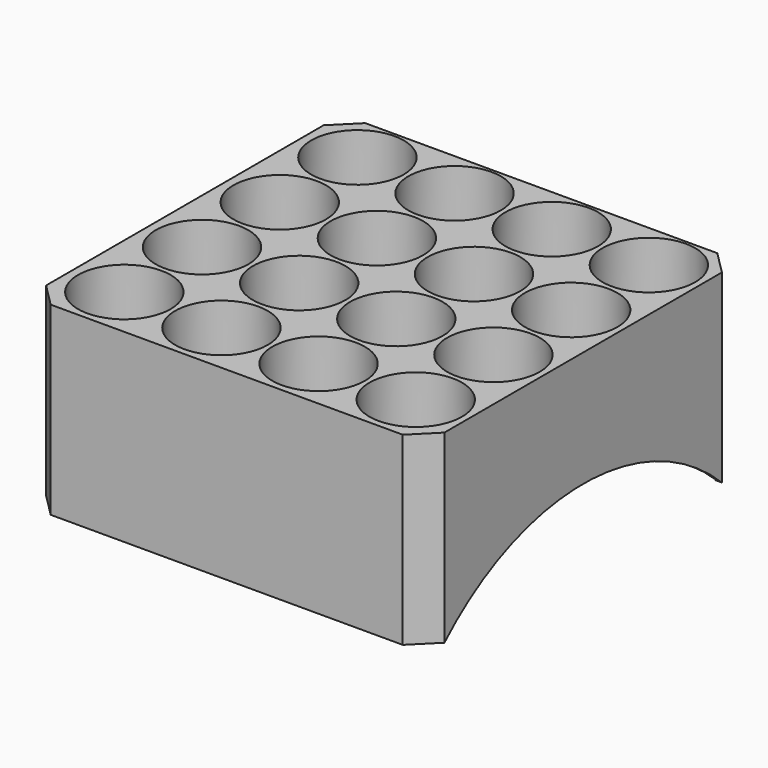
from build123d import *

# Parameters (mm, degrees)
F0_W      = 189
F0_H      = 85
F1_DEPTH  = 40
F2_R      = 10
F3_DEPTH  = 39
F4_W      = 102.8933165297
F4_H      = 85
F5_DEPTH  = 40.001
F6_SIZE   = 5
F8_DEPTH  = 25
F10_DEPTH = 86.1076834703


# Not quite as in the source:
# - a feature names something its author has since deleted; it is built from what else it names


with BuildPart() as f1:
    # F0 (on Top) → F1 (new body)
    with BuildSketch(Plane.XY):
        Rectangle(F0_W, F0_H)
    extrude(amount=F1_DEPTH)

    # F2 (on face) → F3 (cut)
    with BuildSketch(Plane.XY.offset(40)):
        with Locations((-82.6875, 31.875)):
            Circle(F2_R)
        with Locations((-61.6875, 31.875)):
            Circle(F2_R)
        with Locations((-40.6875, 31.875)):
            Circle(F2_R)
        with Locations((-19.6875, 31.875)):
            Circle(F2_R)
        with Locations((-19.6875, 10.875)):
            Circle(F2_R)
        with Locations((-40.6875, 10.875)):
            Circle(F2_R)
        with Locations((-61.6875, 10.875)):
            Circle(F2_R)
        with Locations((-82.6875, 10.875)):
            Circle(F2_R)
        with Locations((-82.6875, -10.125)):
            Circle(F2_R)
        with Locations((-61.6875, -10.125)):
            Circle(F2_R)
        with Locations((-40.6875, -10.125)):
            Circle(F2_R)
        with Locations((-19.6875, -10.125)):
            Circle(F2_R)
        with Locations((-19.6875, -31.125)):
            Circle(F2_R)
        with Locations((-40.6875, -31.125)):
            Circle(F2_R)
        with Locations((-61.6875, -31.125)):
            Circle(F2_R)
        with Locations((-82.6875, -31.125)):
            Circle(F2_R)
    extrude(amount=-F3_DEPTH, mode=Mode.SUBTRACT)

    # F4 (on face) → F5 (cut, through all)
    with BuildSketch(Plane.XY.offset(40)):
        with Locations((43.0533417352, 0)):
            Rectangle(F4_W, F4_H)
    extrude(amount=-F5_DEPTH, mode=Mode.SUBTRACT)

    # F6
    f6_edges = [f1.edges().sort_by_distance(p)[0] for p in [
        (-94.5, 42.5, 20),
        (-8.393317, 42.5, 20),
        (-8.393317, -42.5, 20),
        (-94.5, -42.5, 20),
    ]]
    chamfer(f6_edges, length=F6_SIZE)

    # F7 (on face) → F8 (cut)
    with BuildSketch(Plane(origin=(0, 0, 0), x_dir=(1, 0, 0), z_dir=(0, 0, -1))):
        Polygon((-9.3933165297, -37.0857864376), (-9.3933165297, 37.0857864376), (-13.8075300921, 41.5), (-89.0857864376, 41.5), (-93.5, 37.0857864376), (-93.5, -37.0857864376), (-89.0857864376, -41.5), (-13.8075300921, -41.5), align=None)
    extrude(amount=-F8_DEPTH, mode=Mode.SUBTRACT)

    # F9 (on face) → F10 (cut, through all)
    with BuildSketch(Plane.YZ.offset(-8.3933165297)):
        with BuildLine():
            Line((-37.5, 0), (37.5, 0))
            ThreePointArc((37.5, 0), (0, 15), (-37.5, 0))
        make_face()
    extrude(amount=-F10_DEPTH, mode=Mode.SUBTRACT)


solid = f1.part
